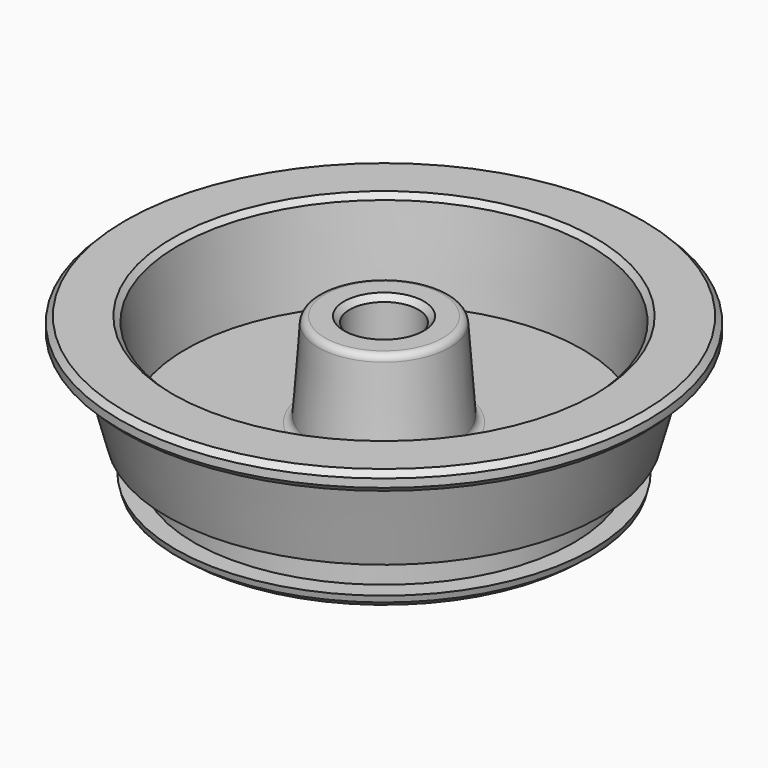
from build123d import *

# Parameters (mm, degrees)
F3_R     = 0.5
F4_R     = 11
F5_DEPTH = 1
F6_SIZE  = 0.5


# Not quite as in the source:
# - a fillet or chamfer that OpenCascade refuses, or shapes differently, is made with other operations: its cross-section is extruded or revolved along the edge and cut away or added


with BuildPart() as f1:
    # F0 (on Front) → F1 (revolve)
    with BuildSketch(Plane.XZ):
        Polygon((4.75, 11), (2.5, 11), (2.5, 0), (14.8776877527, 0), (15.1418584287, 0.9858983849), (13.8, 0.9858983849), (13.8, 3.2858983849), (15.7581415713, 3.2858983849), (17.45, 9.6), (19.2, 9.6), (19.2, 11), (15, 11), (14.405077088, 4.2), (5.25, 4.2), align=None)
    revolve(axis=Axis((0, 0, 5.5), (0, 0, 1)))

    # F2: chamfer of 0.4 on 4 edges, made by hand

    # F2_s1 → F2_t2 (revolve, cut)
    with BuildSketch(Plane.XZ):
        Polygon((2.9, 11), (2.5, 10.6), (2.5, 11), align=None)
    revolve(axis=Axis((0, 0, 11), (0, 0, 1)), mode=Mode.SUBTRACT)

    # F2_s3 → F2_t4 (revolve, cut)
    with BuildSketch(Plane.XZ):
        Polygon((19.2, 10.6), (18.8, 11), (19.2, 11), align=None)
    revolve(axis=Axis((0, 0, 11), (0, 0, 1)), mode=Mode.SUBTRACT)

    # F2_s5 → F2_t6 (revolve, cut)
    with BuildSketch(Plane.XZ):
        Polygon((15.3665324696, 11), (14.9680545904, 10.6348622971), (15, 11), align=None)
    revolve(axis=Axis((0, 0, 11), (0, 0, 1)), mode=Mode.SUBTRACT)

    # F2_s7 → F2_t8 (revolve, cut)
    with BuildSketch(Plane.XZ):
        Polygon((18.8, 9.6), (19.2, 10), (19.2, 9.6), align=None)
    revolve(axis=Axis((0, 0, 9.6), (0, 0, 1)), mode=Mode.SUBTRACT)

    # F3
    f3_edges = [f1.edges().sort_by_distance(p)[0] for p in [
        (-5.25, 0, 4.2),
        (-4.75, 0, 11),
        (5, 0, 7.6),
    ]]
    fillet(f3_edges, radius=F3_R)

    # F4 (on face) → F5 (cut)
    with BuildSketch(Plane(origin=(0, 0, 0), x_dir=(1, 0, 0), z_dir=(0, 0, -1))):
        Circle(F4_R)
    extrude(amount=-F5_DEPTH, mode=Mode.SUBTRACT)

    # F6
    f6_edges = [f1.edges().sort_by_distance(p)[0] for p in [
        (-14.877688, 0, 0),
    ]]
    chamfer(f6_edges, length=F6_SIZE)


solid = f1.part
